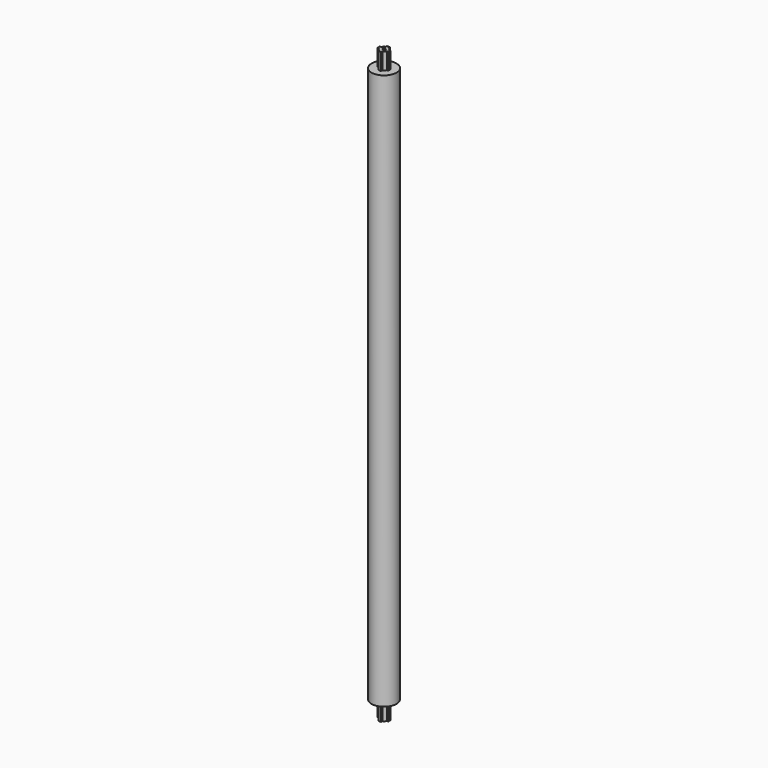
from build123d import *

# Parameters (mm, degrees)
F0_R     = 22.5
F1_DEPTH = 1000
F4_DEPTH = 31
F5_R     = 2.5
F6_DEPTH = 40
F7_DEPTH = 30
F8_R     = 2.5
F9_DEPTH = 30


with BuildPart() as f1:
    # F0 (on Top) → F1 (new body)
    with BuildSketch(Plane.XY):
        Circle(F0_R)
    extrude(amount=F1_DEPTH)

    # F3 (on face) → F4 (join)
    with BuildSketch(Plane(origin=(0, 0, 0), x_dir=(1, 0, 0), z_dir=(0, 0, -1))):
        with BuildLine():
            ThreePointArc((7.0710678119, 2.5), (7.3919891974, 1.2682648404), (7.5, 0))
            ThreePointArc((7.5, 0), (7.3919069765, -1.268743966), (7.0707436663, -2.500916633))
            Line((7.0707436663, -2.500916633), (9.7997435124, -2.5))
            Line((9.7997435124, -2.5), (9.7997435124, 0))
            Line((9.7997435124, 0), (9.7997435124, 2.5))
            Line((9.7997435124, 2.5), (7.0710678119, 2.5))
        make_face()
        with BuildLine():
            Line((2.5, -9.7997435124), (2.5, -7.0710678119))
            ThreePointArc((2.5, -7.0710678119), (-0.0004861292, -7.4999999842), (-2.500916633, -7.0707436663))
            Line((-2.500916633, -7.0707436663), (-2.5, -9.7997435124))
            Line((-2.5, -9.7997435124), (0, -9.7997435124))
            Line((0, -9.7997435124), (2.5, -9.7997435124))
        make_face()
        with BuildLine():
            ThreePointArc((-7.0710678119, -2.5), (-7.4999999842, 0.0004861292), (-7.0707436663, 2.500916633))
            Line((-7.0707436663, 2.500916633), (-9.7997435124, 2.5))
            Line((-9.7997435124, 2.5), (-9.7997435124, 0))
            Line((-9.7997435124, 0), (-9.7997435124, -2.5))
            Line((-9.7997435124, -2.5), (-7.0710678119, -2.5))
        make_face()
        with BuildLine():
            ThreePointArc((7.0707436663, -2.500916633), (7.3919069765, -1.268743966), (7.5, 0))
            ThreePointArc((7.5, 0), (7.3919891974, 1.2682648404), (7.0710678119, 2.5))
            ThreePointArc((7.0710678119, 2.5), (5.303644593, 5.3029571025), (2.500916633, 7.0707436663))
            ThreePointArc((2.500916633, 7.0707436663), (0.0004861292, 7.4999999842), (-2.5, 7.0710678119))
            ThreePointArc((-2.5, 7.0710678119), (-5.3029571025, 5.303644593), (-7.0707436663, 2.500916633))
            ThreePointArc((-7.0707436663, 2.500916633), (-7.4999999842, 0.0004861292), (-7.0710678119, -2.5))
            ThreePointArc((-7.0710678119, -2.5), (-5.303644593, -5.3029571025), (-2.500916633, -7.0707436663))
            ThreePointArc((-2.500916633, -7.0707436663), (-0.0004861292, -7.4999999842), (2.5, -7.0710678119))
            ThreePointArc((2.5, -7.0710678119), (5.3029571025, -5.303644593), (7.0707436663, -2.500916633))
        make_face()
        with BuildLine():
            ThreePointArc((-2.5, 7.0710678119), (0.0004861292, 7.4999999842), (2.500916633, 7.0707436663))
            Line((2.500916633, 7.0707436663), (2.5, 9.7997435124))
            Line((2.5, 9.7997435124), (0, 9.7997435124))
            Line((0, 9.7997435124), (-2.5, 9.7997435124))
            Line((-2.5, 9.7997435124), (-2.5, 7.0710678119))
        make_face()
    extrude(amount=F4_DEPTH)

    # F5 (on face) → F6 (cut)
    with BuildSketch(Plane(origin=(0, 0, -31), x_dir=(1, 0, 0), z_dir=(0, 0, -1))):
        Circle(F5_R)
    extrude(amount=-F6_DEPTH, mode=Mode.SUBTRACT)

    # F2 (on face) → F7 (join)
    with BuildSketch(Plane.XY.offset(1000)):
        with BuildLine():
            ThreePointArc((7.0707436663, -2.500916633), (7.3919069765, -1.268743966), (7.5, 0))
            ThreePointArc((7.5, 0), (7.3919891974, 1.2682648404), (7.0710678119, 2.5))
            ThreePointArc((7.0710678119, 2.5), (5.303644593, 5.3029571025), (2.500916633, 7.0707436663))
            ThreePointArc((2.500916633, 7.0707436663), (0.0004861292, 7.4999999842), (-2.5, 7.0710678119))
            ThreePointArc((-2.5, 7.0710678119), (-5.3029571025, 5.303644593), (-7.0707436663, 2.500916633))
            ThreePointArc((-7.0707436663, 2.500916633), (-7.4999999842, 0.0004861292), (-7.0710678119, -2.5))
            ThreePointArc((-7.0710678119, -2.5), (-5.303644593, -5.3029571025), (-2.500916633, -7.0707436663))
            ThreePointArc((-2.500916633, -7.0707436663), (-0.0004861292, -7.4999999842), (2.5, -7.0710678119))
            ThreePointArc((2.5, -7.0710678119), (5.3029571025, -5.303644593), (7.0707436663, -2.500916633))
        make_face()
        with BuildLine():
            ThreePointArc((-7.0710678119, -2.5), (-7.4999999842, 0.0004861292), (-7.0707436663, 2.500916633))
            Line((-7.0707436663, 2.500916633), (-9.7997435124, 2.5))
            Line((-9.7997435124, 2.5), (-9.7997435124, 0))
            Line((-9.7997435124, 0), (-9.7997435124, -2.5))
            Line((-9.7997435124, -2.5), (-7.0710678119, -2.5))
        make_face()
        with BuildLine():
            ThreePointArc((-2.5, 7.0710678119), (0.0004861292, 7.4999999842), (2.500916633, 7.0707436663))
            Line((2.500916633, 7.0707436663), (2.5, 9.7997435124))
            Line((2.5, 9.7997435124), (0, 9.7997435124))
            Line((0, 9.7997435124), (-2.5, 9.7997435124))
            Line((-2.5, 9.7997435124), (-2.5, 7.0710678119))
        make_face()
        with BuildLine():
            ThreePointArc((7.0710678119, 2.5), (7.3919891974, 1.2682648404), (7.5, 0))
            ThreePointArc((7.5, 0), (7.3919069765, -1.268743966), (7.0707436663, -2.500916633))
            Line((7.0707436663, -2.500916633), (9.7997435124, -2.5))
            Line((9.7997435124, -2.5), (9.7997435124, 0))
            Line((9.7997435124, 0), (9.7997435124, 2.5))
            Line((9.7997435124, 2.5), (7.0710678119, 2.5))
        make_face()
        with BuildLine():
            Line((2.5, -9.7997435124), (2.5, -7.0710678119))
            ThreePointArc((2.5, -7.0710678119), (-0.0004861292, -7.4999999842), (-2.500916633, -7.0707436663))
            Line((-2.500916633, -7.0707436663), (-2.5, -9.7997435124))
            Line((-2.5, -9.7997435124), (0, -9.7997435124))
            Line((0, -9.7997435124), (2.5, -9.7997435124))
        make_face()
    extrude(amount=F7_DEPTH)

    # F8 (on face) → F9 (cut)
    with BuildSketch(Plane.XY.offset(1030)):
        Circle(F8_R)
    extrude(amount=-F9_DEPTH, mode=Mode.SUBTRACT)


solid = f1.part
